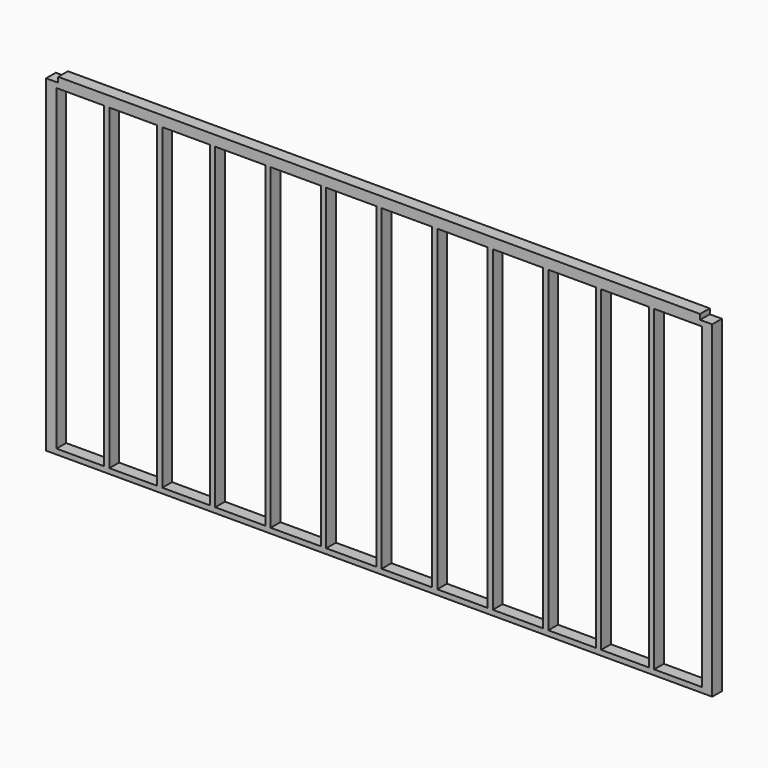
from build123d import *

# Parameters (mm, degrees)
F0_W     = 38.1
F0_H     = 2324.1
F0_W_2   = 4699
F0_H_2   = 38.1
F1_DEPTH = 88.9


# Not quite as in the source:
# - a feature names something its author has since deleted; it is built from what else it names


with BuildPart() as f1:
    # F0 (on Front) → F1 (new body)
    with BuildSketch(Plane.XZ):
        with Locations((19.05, 1200.15)):
            Rectangle(F0_W, F0_H)
        with Locations((57.15, 1200.15)):
            Rectangle(F0_W, F0_H)
        with Locations((444.5, 1200.15)):
            Rectangle(F0_W, F0_H)
        with Locations((831.85, 1200.15)):
            Rectangle(F0_W, F0_H)
        with Locations((1219.2, 1200.15)):
            Rectangle(F0_W, F0_H)
        with Locations((2032, 1200.15)):
            Rectangle(F0_W, F0_H)
        with Locations((4819.65, 1200.15)):
            Rectangle(F0_W, F0_H)
        with Locations((4857.75, 1200.15)):
            Rectangle(F0_W, F0_H)
        Polygon((0, 2400.3), (0, 2362.2), (38.1, 2362.2), (76.2, 2362.2), (425.45, 2362.2), (463.55, 2362.2), (812.8, 2362.2), (850.9, 2362.2), (1200.15, 2362.2), (1238.25, 2362.2), (1606.55, 2362.2), (1644.65, 2362.2), (2012.95, 2362.2), (2051.05, 2362.2), (2419.35, 2362.2), (2457.45, 2362.2), (2825.75, 2362.2), (2863.85, 2362.2), (3232.15, 2362.2), (3270.25, 2362.2), (3638.55, 2362.2), (3676.65, 2362.2), (4025.9, 2362.2), (4064, 2362.2), (4413.25, 2362.2), (4451.35, 2362.2), (4800.6, 2362.2), (4838.7, 2362.2), (4876.8, 2362.2), (4876.8, 2400.3), (4787.9, 2400.3), (88.9, 2400.3), align=None)
        with Locations((2438.4, 2419.35)):
            Rectangle(F0_W_2, F0_H_2)
        Polygon((0, 38.1), (0, 0), (4876.8, 0), (4876.8, 38.1), (4838.7, 38.1), (4800.6, 38.1), (4451.35, 38.1), (4413.25, 38.1), (4064, 38.1), (4025.9, 38.1), (3676.65, 38.1), (3638.55, 38.1), (3270.25, 38.1), (3232.15, 38.1), (2863.85, 38.1), (2825.75, 38.1), (2457.45, 38.1), (2419.35, 38.1), (2051.05, 38.1), (2012.95, 38.1), (1644.65, 38.1), (1606.55, 38.1), (1238.25, 38.1), (1200.15, 38.1), (850.9, 38.1), (812.8, 38.1), (463.55, 38.1), (425.45, 38.1), (76.2, 38.1), (38.1, 38.1), align=None)
        with Locations((1625.6, 1200.15)):
            Rectangle(F0_W, F0_H)
        with Locations((2438.4, 1200.15)):
            Rectangle(F0_W, F0_H)
        with Locations((2844.8, 1200.15)):
            Rectangle(F0_W, F0_H)
        with Locations((3251.2, 1200.15)):
            Rectangle(F0_W, F0_H)
        with Locations((3657.6, 1200.15)):
            Rectangle(F0_W, F0_H)
        with Locations((4044.95, 1200.15)):
            Rectangle(F0_W, F0_H)
        with Locations((4432.3, 1200.15)):
            Rectangle(F0_W, F0_H)
    extrude(amount=F1_DEPTH)


solid = f1.part
